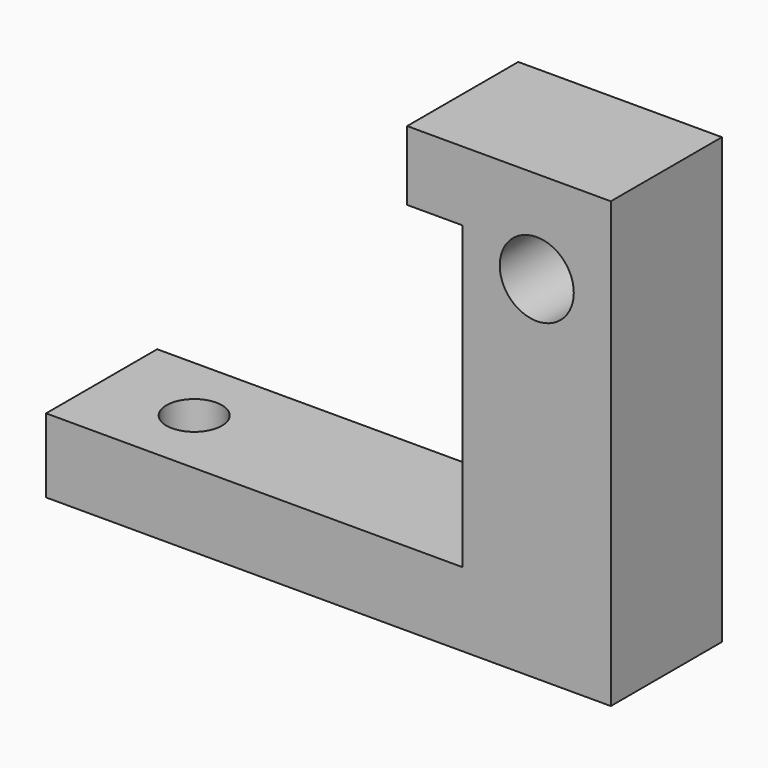
from build123d import *

# Parameters (mm, degrees)
F0_W     = 45
F0_H     = 8
F0_W_2   = 16
F0_R     = 4
F0_H_2   = 2
F1_DEPTH = 15
F2_R     = 3
F3_DEPTH = 55.5


# Not quite as in the source:
# - a feature names something its author has since deleted; it is built from what else it names


with BuildPart() as f1:
    # F0 (on Front) → F1 (new body)
    with BuildSketch(Plane.XZ):
        with Locations((22.5, 4)):
            Rectangle(F0_W, F0_H)
        with Locations((53, 4)):
            Rectangle(F0_W_2, F0_H)
        Polygon((45, 40.5), (45, 8), (61, 8), (61, 46), (45, 46), align=None)
        with Locations((53, 38)):
            Circle(F0_R, mode=Mode.SUBTRACT)
        Polygon((39, 40.5), (45, 40.5), (45, 46), (45, 48), (39, 48), align=None)
        with Locations((53, 47)):
            Rectangle(F0_W_2, F0_H_2)
    extrude(amount=F1_DEPTH)

    # F2 (on face) → F3 (cut, symmetric)
    with BuildSketch(Plane.XY.offset(8)):
        with Locations((10, -7.5)):
            Circle(F2_R)
    extrude(amount=F3_DEPTH, both=True, mode=Mode.SUBTRACT)


solid = f1.part
